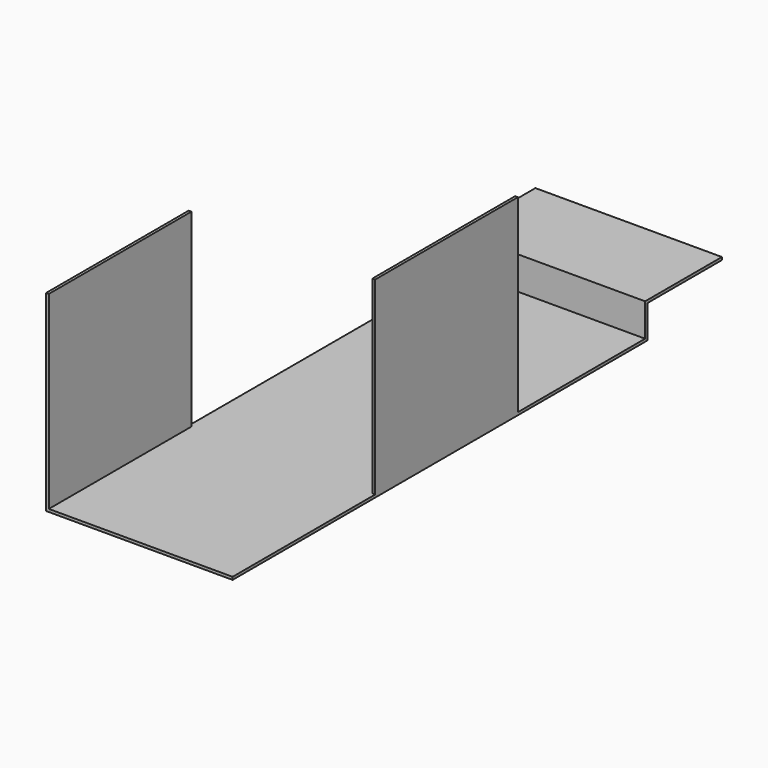
from build123d import *

# Parameters (mm, degrees)
F0_W     = 68
F0_H     = 188
F1_DEPTH = 1
F0_H_2   = 35
F2_DEPTH = 13
F3_W     = 68
F3_H     = 34
F4_DEPTH = 12
F5_W     = 65
F5_H     = 69
F6_DEPTH = 1
F7_W     = 65
F7_H     = 69
F8_DEPTH = 1


# Not quite as in the source:
# - a feature names something its author has since deleted; it is built from what else it names


with BuildPart() as f1:
    # F0 (on Top) → F1 (new body)
    with BuildSketch(Plane.XY):
        with Locations((145.9408301511, 2.5440129265)):
            Rectangle(F0_W, F0_H)
    extrude(amount=F1_DEPTH)

    # F0 (on Top) → F2 (join)
    with BuildSketch(Plane.XY):
        with Locations((145.9408301511, 114.0440129265)):
            Rectangle(F0_W, F0_H_2)
    extrude(amount=F2_DEPTH)

    # F3 (on face) → F4 (cut)
    with BuildSketch(Plane(origin=(0, 0, 0), x_dir=(1, 0, 0), z_dir=(0, 0, -1))):
        with Locations((145.9408301511, -114.5440129265)):
            Rectangle(F3_W, F3_H)
    extrude(amount=-F4_DEPTH, mode=Mode.SUBTRACT)

    # F5 (on face) → F6 (join)
    with BuildSketch(Plane.YZ.offset(179.9408301511)):
        with Locations((6.0440129265, 35.5)):
            Rectangle(F5_W, F5_H)
    extrude(amount=-F6_DEPTH)

    # F7 (on face) → F8 (join)
    with BuildSketch(Plane(origin=(111.9408301511, 0, 0), x_dir=(0, -1, 0), z_dir=(-1, 0, 0))):
        with Locations((58.9559870735, 35.5)):
            Rectangle(F7_W, F7_H)
    extrude(amount=-F8_DEPTH)


with BuildPart() as f1_1:
    # F9: moved
    add(f1.part.moved(Location((-146.441, 0, 0))))


solid = f1_1.part
